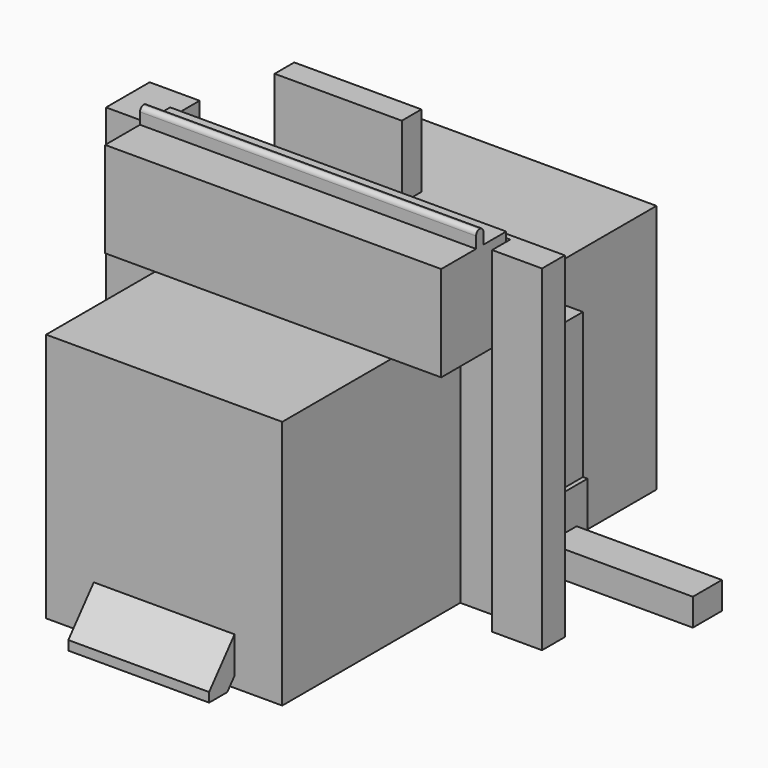
from build123d import *

# Parameters (mm, degrees)
F0_W      = 155
F0_H      = 52
F1_DEPTH  = 65
F2_SIZE2  = 41.7113757408
F2_SIZE   = 35
F3_SIZE2  = 47.6701437038
F3_SIZE   = 40
F4_W      = 60.4387485981
F4_H      = 52
F5_DEPTH  = 155.001
F6_W      = 260
F6_H      = 75
F7_DEPTH  = 435
F8_W      = 6.3
F8_H      = 370
F9_DEPTH  = 55
F10_W     = 6.3
F10_H     = 40.3
F11_DEPTH = 260
F12_W     = 55
F12_H     = 370
F13_DEPTH = 6.3
F14_W     = 95
F14_H     = 115
F15_DEPTH = 55
F16_W     = 100
F16_H     = 230
F17_DEPTH = 55
F18_W     = 260
F18_H     = 75
F19_DEPTH = 80
F20_W     = 40
F20_H     = 30
F21_DEPTH = 60
F22_W     = 60
F22_H     = 370
F23_DEPTH = 55
F24_W     = 60
F24_H     = 370
F25_DEPTH = 55
F27_DEPTH = 55
F29_DEPTH = 200
F30_W     = 370
F30_H     = 105
F31_DEPTH = 95
F32_W     = 370
F32_H     = 10
F33_DEPTH = 17.5
F34_R     = 4.99999
F35_W     = 370
F35_H     = 5.5
F36_DEPTH = 105
F37_W     = 140
F37_H     = 27
F38_DEPTH = 80
F39_DEPTH = 100
F40_W     = 100
F40_H     = 160
F41_DEPTH = 5


# Not quite as in the source:
# - a fillet or chamfer is up to 0.001 mm smaller than in the source, because OpenCascade refuses the exact size


with BuildPart() as f1:
    # F0 (on Front) → F1 (new body)
    with BuildSketch(Plane.XZ):
        with Locations((0, 26)):
            Rectangle(F0_W, F0_H)
    extrude(amount=-F1_DEPTH)

    # F2
    f2_edges = [f1.edges().sort_by_distance(p)[0] for p in [
        (0, 0, 52),
    ]]
    f2_side = f1.faces().sort_by_distance((0, 32.5, 52))[0]
    chamfer(f2_edges, length=F2_SIZE, length2=F2_SIZE2, reference=f2_side)

    # F3
    f3_edges = [f1.edges().sort_by_distance(p)[0] for p in [
        (0, 65, 0),
    ]]
    f3_side = f1.faces().sort_by_distance((0, 32.5, 0))[0]
    chamfer(f3_edges, length=F3_SIZE, length2=F3_SIZE2, reference=f3_side)

    # F4 (on face) → F5 (cut, through all)
    with BuildSketch(Plane(origin=(-77.5, 0, 0), x_dir=(0, -1, 0), z_dir=(-1, 0, 0))):
        with Locations((-65.219374299, 26)):
            Rectangle(F4_W, F4_H)
    extrude(amount=-F5_DEPTH, mode=Mode.SUBTRACT)

    # F6 (on face) → F7 (join)
    with BuildSketch(Plane(origin=(0, 35, 0), x_dir=(-1, 0, 0), z_dir=(0, 1, 0))):
        with Locations((0, 37.5)):
            Rectangle(F6_W, F6_H)
    extrude(amount=F7_DEPTH)

    # F8 (on face) → F9 (join)
    with BuildSketch(Plane(origin=(-130, 0, 0), x_dir=(0, -1, 0), z_dir=(-1, 0, 0))):
        with Locations((-283.15, 185)):
            Rectangle(F8_W, F8_H)
    extrude(amount=F9_DEPTH)

    # F10 (on face) → F11 (join)
    with BuildSketch(Plane.YZ.offset(-130)):
        with Locations((283.15, 349.85)):
            Rectangle(F10_W, F10_H)
    extrude(amount=F11_DEPTH)

    # F12 (on face) → F13 (join)
    with BuildSketch(Plane.XZ.offset(-280)):
        with Locations((157.5, 185)):
            Rectangle(F12_W, F12_H)
    extrude(amount=-F13_DEPTH)

    # F14 (on face) → F15 (join)
    with BuildSketch(Plane(origin=(-185, 0, 0), x_dir=(0, -1, 0), z_dir=(-1, 0, 0))):
        with Locations((-333.8, 122.5)):
            Rectangle(F14_W, F14_H)
    extrude(amount=-F15_DEPTH)

    # F16 (on face) → F17 (join)
    with BuildSketch(Plane.YZ.offset(185)):
        with Locations((336.3, 140)):
            Rectangle(F16_W, F16_H)
    extrude(amount=-F17_DEPTH)

    # F18 (on face) → F19 (join)
    with BuildSketch(Plane(origin=(0, 470, 0), x_dir=(-1, 0, 0), z_dir=(0, 1, 0))):
        with Locations((0, 37.5)):
            Rectangle(F18_W, F18_H)
    extrude(amount=F19_DEPTH)

    # F20 (on face) → F21 (join)
    with BuildSketch(Plane.YZ.offset(185)):
        with Locations((351.3, 40)):
            Rectangle(F20_W, F20_H)
    extrude(amount=F21_DEPTH)

    # F22 (on face) → F23 (join)
    with BuildSketch(Plane(origin=(-185, 0, 0), x_dir=(0, -1, 0), z_dir=(-1, 0, 0))):
        with Locations((-285, 185)):
            Rectangle(F22_W, F22_H)
    extrude(amount=F23_DEPTH)

    # F24 (on face) → F25 (join)
    with BuildSketch(Plane.YZ.offset(185)):
        with Locations((285, 185)):
            Rectangle(F24_W, F24_H)
    extrude(amount=F25_DEPTH)

    # F26 (on face) → F27 (cut)
    with BuildSketch(Plane.YZ.offset(240)):
        Polygon((315, 0), (315, 25), (315, 255), (315, 370), (286.3, 370), (286.3, 255), (286.3, 0), align=None)
    extrude(amount=-F27_DEPTH, mode=Mode.SUBTRACT)

    # F28 (on face) → F29 (join)
    with BuildSketch(Plane.XY.offset(75)):
        Polygon((-130, 381.3), (-130, 280), (-130, 35), (130, 35), (130, 280), (130, 386.3), (130, 550), (-130, 550), align=None)
    extrude(amount=F29_DEPTH)

    # F39 (add): a face of the model
    f39_faces = [f1.faces().sort_by_distance(p)[0] for p in [
        (245, 351.3, 40),
    ]]
    extrude(f39_faces, amount=F39_DEPTH)

    # F40 (on face) → F41 (cut)
    with BuildSketch(Plane.YZ.offset(185)):
        with Locations((336.3, 175)):
            Rectangle(F40_W, F40_H)
    extrude(amount=-F41_DEPTH, mode=Mode.SUBTRACT)


with BuildPart() as f31:
    # F30 (on face) → F31 (new body)
    with BuildSketch(Plane.XZ.offset(-280)):
        with Locations((0, 327.5)):
            Rectangle(F30_W, F30_H)
    extrude(amount=F31_DEPTH)

    # F32 (on face) → F33 (join)
    with BuildSketch(Plane.XY.offset(380)):
        with Locations((0, 238)):
            Rectangle(F32_W, F32_H)
    extrude(amount=F33_DEPTH)

    # F34 (radius 5 in the source; OpenCascade refuses exactly that, so slightly less here)
    f34_edges = [f31.edges().sort_by_distance(p)[0] for p in [
        (0, 233, 397.5),
        (0, 243, 397.5),
    ]]
    fillet(f34_edges, radius=F34_R)

    # F35 (on face) → F36 (cut)
    with BuildSketch(Plane.XY.offset(380)):
        with Locations((0, 277.25)):
            Rectangle(F35_W, F35_H)
    extrude(amount=-F36_DEPTH, mode=Mode.SUBTRACT)


with BuildPart() as f38:
    # F37 (on face) → F38 (new body)
    with BuildSketch(Plane.XY.offset(370)):
        with Locations((0, 288)):
            Rectangle(F37_W, F37_H)
    extrude(amount=F38_DEPTH)


solid = Compound([f1.part, f31.part, f38.part])
